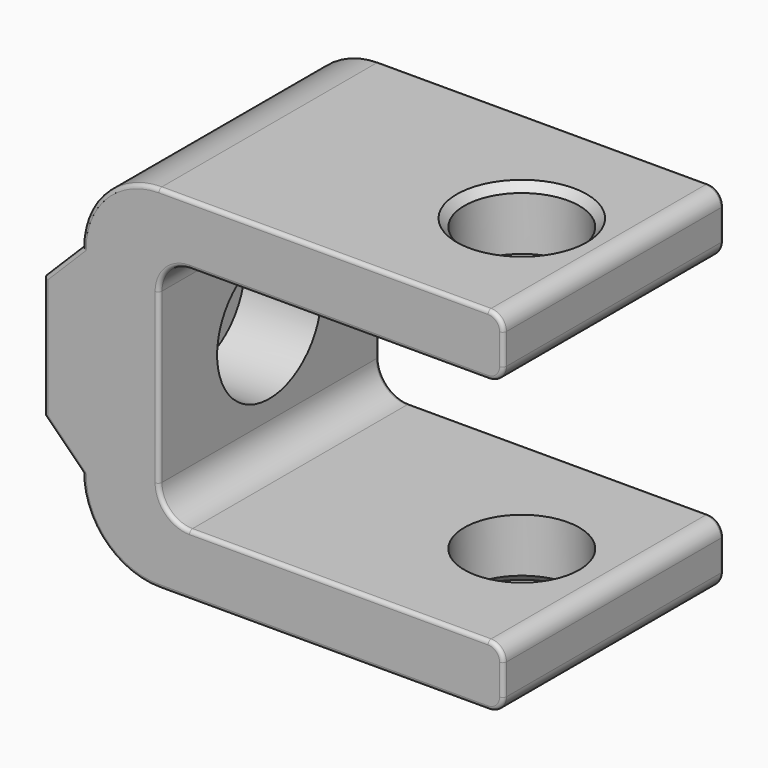
from build123d import *

# Parameters (mm, degrees)
F1_DEPTH       = 18
F2_R           = 7.5
F3_DEPTH       = 46.001
F5_D           = 10
F5_CBORE_D     = 17
F5_CBORE_DEPTH = 10
F6_SIZE2       = 1
F6_SIZE        = 1
F7_R           = 0.5


with BuildPart() as f1:
    # F0 (on Front) → F1 (new body, symmetric)
    with BuildSketch(Plane.XZ):
        with BuildLine():
            ThreePointArc((30, 21), (29.4142135624, 22.4142135624), (28, 23))
            Line((28, 23), (-15, 23))
            ThreePointArc((-15, 23), (-22.0710678119, 20.0710678119), (-25, 13))
            Line((-25, 13), (-30, 8))
            Line((-30, 8), (-30, -8))
            Line((-30, -8), (-25, -13))
            ThreePointArc((-25, -13), (-22.0710678119, -20.0710678119), (-15, -23))
            Line((-15, -23), (28, -23))
            ThreePointArc((28, -23), (29.4142135624, -22.4142135624), (30, -21))
            Line((30, -21), (30, -17))
            ThreePointArc((30, -17), (29.4142135624, -15.5857864376), (28, -15))
            Line((28, -15), (-11, -15))
            ThreePointArc((-11, -15), (-13.8284271247, -13.8284271247), (-15, -11))
            Line((-15, -11), (-15, 11))
            ThreePointArc((-15, 11), (-13.8284271247, 13.8284271247), (-11, 15))
            Line((-11, 15), (28, 15))
            ThreePointArc((28, 15), (29.4142135624, 15.5857864376), (30, 17))
            Line((30, 17), (30, 21))
        make_face()
    extrude(amount=F1_DEPTH, both=True)

    # F2 (on face) → F3 (cut, through all)
    with BuildSketch(Plane.XY.offset(23)):
        with Locations((18, 0)):
            Circle(F2_R)
    extrude(amount=-F3_DEPTH, mode=Mode.SUBTRACT)

    # F5 (through all)
    with Locations(Plane.YZ.offset(-15)):
        with Locations((0, 0)):
            CounterBoreHole(F5_D / 2, F5_CBORE_D / 2, F5_CBORE_DEPTH)

    # F6
    f6_edges = [f1.edges().sort_by_distance(p)[0] for p in [
        (10.5, 0, -23),
        (10.5, 0, 23),
        (-30, -5, 0),
    ]]
    chamfer(f6_edges, length=F6_SIZE, length2=F6_SIZE2)

    # F7
    f7_edges = [f1.edges().sort_by_distance(p)[0] for p in [
        (29.414214, 18, 22.414214),
        (6.5, 18, 23),
        (-22.071068, 18, 20.071068),
        (-27.5, 18, 10.5),
        (-30, 18, 0),
        (-27.5, 18, -10.5),
        (-22.071068, 18, -20.071068),
        (6.5, 18, -23),
        (29.414214, 18, -22.414214),
        (30, 18, -19),
        (29.414214, 18, -15.585786),
        (8.5, 18, -15),
        (-13.828427, 18, -13.828427),
        (-15, 18, 0),
        (-13.828427, 18, 13.828427),
        (8.5, 18, 15),
        (29.414214, 18, 15.585786),
        (30, 18, 19),
        (29.414214, -18, 22.414214),
        (6.5, -18, 23),
        (-22.071068, -18, 20.071068),
        (-27.5, -18, 10.5),
        (-30, -18, 0),
        (-27.5, -18, -10.5),
        (-22.071068, -18, -20.071068),
        (6.5, -18, -23),
        (29.414214, -18, -22.414214),
        (30, -18, -19),
        (29.414214, -18, -15.585786),
        (8.5, -18, -15),
        (-13.828427, -18, -13.828427),
        (-15, -18, 0),
        (-13.828427, -18, 13.828427),
        (8.5, -18, 15),
        (29.414214, -18, 15.585786),
        (30, -18, 19),
    ]]
    fillet(f7_edges, radius=F7_R)


solid = f1.part
